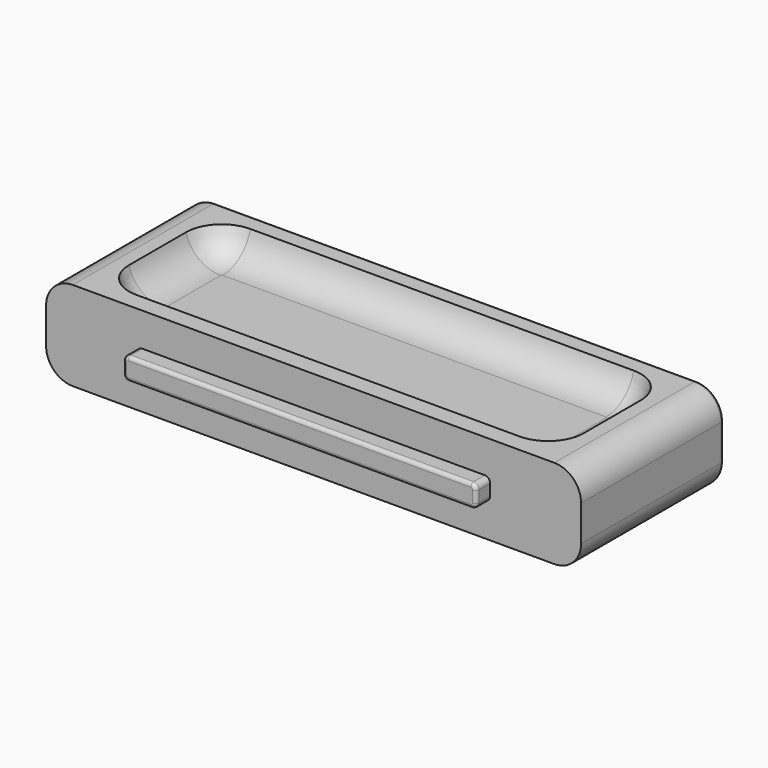
from build123d import *

# Parameters (mm, degrees)
F0_W          = 76.2
F0_H          = 12.7
F1_DEPTH      = 25.4
F2_W          = 50.292
F2_H          = 3.1496
F3_DEPTH      = 2.4892
F4_R          = 0.762
F5_R          = 0.508
F6_R          = 3.81
F7_W          = 64.77
F7_H          = 20.32
F8_DEPTH      = 3.81
F9_R          = 5.08
F10_T1_DEPTH  = 54.61
F10_T3_DEPTH  = 10.16
F10_T6_ANGLE  = 90
F10_T8_ANGLE  = 90
F10_T10_ANGLE = 90
F10_T12_ANGLE = 90
F11_W         = 64.77
F11_H         = 20.32
F12_DEPTH     = 3.81
F13_R         = 5.08
F14_T1_DEPTH  = 54.61
F14_T3_DEPTH  = 10.16
F14_T6_ANGLE  = 90
F14_T8_ANGLE  = 90
F14_T10_ANGLE = 90
F14_T12_ANGLE = 90
F15_R         = 0.508


# Not quite as in the source:
# - a fillet or chamfer that OpenCascade refuses, or shapes differently, is made with other operations: its cross-section is extruded or revolved along the edge and cut away or added


with BuildPart() as f1:
    # F0 (on Front) → F1 (new body)
    with BuildSketch(Plane.XZ):
        Rectangle(F0_W, F0_H)
    extrude(amount=F1_DEPTH)

    # F2 (on face) → F3 (join)
    with BuildSketch(Plane.XZ.offset(25.4)):
        Rectangle(F2_W, F2_H)
    extrude(amount=F3_DEPTH)

    # F4
    f4_edges = [f1.edges().sort_by_distance(p)[0] for p in [
        (-25.146, -26.6446, 1.5748),
        (-25.146, -26.6446, -1.5748),
        (25.146, -26.6446, 1.5748),
        (25.146, -26.6446, -1.5748),
    ]]
    fillet(f4_edges, radius=F4_R)

    # F5
    f5_edges = [f1.edges().sort_by_distance(p)[0] for p in [
        (0, -27.8892, 1.5748),
        (24.922815, -27.8892, 1.351615),
        (-24.922815, -27.8892, 1.351615),
        (25.146, -27.8892, 0),
        (-25.146, -27.8892, 0),
        (24.922815, -27.8892, -1.351615),
        (-24.922815, -27.8892, -1.351615),
        (0, -27.8892, -1.5748),
    ]]
    fillet(f5_edges, radius=F5_R)

    # F6
    f6_edges = [f1.edges().sort_by_distance(p)[0] for p in [
        (38.1, -12.7, 6.35),
        (38.1, -12.7, -6.35),
        (-38.1, -12.7, 6.35),
        (-38.1, -12.7, -6.35),
    ]]
    fillet(f6_edges, radius=F6_R)

    # F7 (on face) → F8 (cut)
    with BuildSketch(Plane.XY.offset(6.35)):
        with Locations((0, -12.7)):
            Rectangle(F7_W, F7_H)
    extrude(amount=-F8_DEPTH, mode=Mode.SUBTRACT)

    # F9
    f9_edges = [f1.edges().sort_by_distance(p)[0] for p in [
        (-32.385, -2.54, 4.445),
        (-32.385, -22.86, 4.445),
        (32.385, -2.54, 4.445),
        (32.385, -22.86, 4.445),
    ]]
    fillet(f9_edges, radius=F9_R)

    # F10: fillet of radius 5.08 on 1 edges, made by hand

    # F10_s2 → F10_t1 (join)
    with BuildSketch(Plane.YZ.offset(-27.305)):
        with BuildLine():
            ThreePointArc((-2.54, 6.35), (-4.3478368763, 3.6039073716), (-7.4586888497, 2.54))
            Line((-7.4586888497, 2.54), (-2.54, 2.54))
            Line((-2.54, 2.54), (-2.54, 6.35))
        make_face()
        with BuildLine():
            ThreePointArc((-22.86, 6.35), (-21.0521631237, 3.6039073716), (-17.9413111503, 2.54))
            Line((-17.9413111503, 2.54), (-22.86, 2.54))
            Line((-22.86, 2.54), (-22.86, 6.35))
        make_face()
    extrude(amount=F10_T1_DEPTH)

    # F10_s4 → F10_t3 (join)
    with BuildSketch(Plane.XZ.offset(7.62)):
        with BuildLine():
            ThreePointArc((-32.385, 6.35), (-30.5771631237, 3.6039073716), (-27.4663111503, 2.54))
            Line((-27.4663111503, 2.54), (-32.385, 2.54))
            Line((-32.385, 2.54), (-32.385, 6.35))
        make_face()
        with BuildLine():
            ThreePointArc((32.385, 6.35), (30.5771631237, 3.6039073716), (27.4663111503, 2.54))
            Line((27.4663111503, 2.54), (32.385, 2.54))
            Line((32.385, 2.54), (32.385, 6.35))
        make_face()
    extrude(amount=F10_T3_DEPTH)

    # F10_s5 → F10_t6 (revolve)
    with BuildSketch(Plane.XZ.offset(7.62)):
        with BuildLine():
            ThreePointArc((32.385, 6.35), (30.5771631237, 3.6039073716), (27.4663111503, 2.54))
            Line((27.4663111503, 2.54), (32.385, 2.54))
            Line((32.385, 2.54), (32.385, 6.35))
        make_face()
    revolve(axis=Axis((27.305, -7.62, 2.54), (0, 0, 1)), revolution_arc=F10_T6_ANGLE)

    # F10_s7 → F10_t8 (revolve)
    with BuildSketch(Plane.XZ.offset(7.62)):
        with BuildLine():
            ThreePointArc((-32.385, 6.35), (-30.5771631237, 3.6039073716), (-27.4663111503, 2.54))
            Line((-27.4663111503, 2.54), (-32.385, 2.54))
            Line((-32.385, 2.54), (-32.385, 6.35))
        make_face()
    revolve(axis=Axis((-27.305, -7.62, 2.54), (0, 0, -1)), revolution_arc=F10_T8_ANGLE)

    # F10_s9 → F10_t10 (revolve)
    with BuildSketch(Plane.YZ.offset(-27.305)):
        with BuildLine():
            ThreePointArc((-22.86, 6.35), (-21.0521631237, 3.6039073716), (-17.9413111503, 2.54))
            Line((-17.9413111503, 2.54), (-22.86, 2.54))
            Line((-22.86, 2.54), (-22.86, 6.35))
        make_face()
    revolve(axis=Axis((-27.305, -17.78, 2.54), (0, 0, -1)), revolution_arc=F10_T10_ANGLE)

    # F10_s11 → F10_t12 (revolve)
    with BuildSketch(Plane.XZ.offset(17.78)):
        with BuildLine():
            ThreePointArc((32.385, 6.35), (30.5771631237, 3.6039073716), (27.4663111503, 2.54))
            Line((27.4663111503, 2.54), (32.385, 2.54))
            Line((32.385, 2.54), (32.385, 6.35))
        make_face()
    revolve(axis=Axis((27.305, -17.78, 2.54), (0, 0, -1)), revolution_arc=F10_T12_ANGLE)

    # F11 (on face) → F12 (cut)
    with BuildSketch(Plane(origin=(0, 0, -6.35), x_dir=(1, 0, 0), z_dir=(0, 0, -1))):
        with Locations((0, 12.7)):
            Rectangle(F11_W, F11_H)
    extrude(amount=-F12_DEPTH, mode=Mode.SUBTRACT)

    # F13
    f13_edges = [f1.edges().sort_by_distance(p)[0] for p in [
        (32.385, -22.86, -4.445),
        (32.385, -2.54, -4.445),
        (-32.385, -22.86, -4.445),
        (-32.385, -2.54, -4.445),
    ]]
    fillet(f13_edges, radius=F13_R)

    # F14: fillet of radius 5.08 on 1 edges, made by hand

    # F14_s2 → F14_t1 (join)
    with BuildSketch(Plane.YZ.offset(-27.305)):
        with BuildLine():
            ThreePointArc((-22.86, -6.35), (-21.0521631237, -3.6039073716), (-17.9413111503, -2.54))
            Line((-17.9413111503, -2.54), (-22.86, -2.54))
            Line((-22.86, -2.54), (-22.86, -6.35))
        make_face()
        with BuildLine():
            ThreePointArc((-2.54, -6.35), (-4.3478368763, -3.6039073716), (-7.4586888497, -2.54))
            Line((-7.4586888497, -2.54), (-2.54, -2.54))
            Line((-2.54, -2.54), (-2.54, -6.35))
        make_face()
    extrude(amount=F14_T1_DEPTH)

    # F14_s4 → F14_t3 (join)
    with BuildSketch(Plane.XZ.offset(7.62)):
        with BuildLine():
            ThreePointArc((32.385, -6.35), (30.5771631237, -3.6039073716), (27.4663111503, -2.54))
            Line((27.4663111503, -2.54), (32.385, -2.54))
            Line((32.385, -2.54), (32.385, -6.35))
        make_face()
        with BuildLine():
            ThreePointArc((-32.385, -6.35), (-30.5771631237, -3.6039073716), (-27.4663111503, -2.54))
            Line((-27.4663111503, -2.54), (-32.385, -2.54))
            Line((-32.385, -2.54), (-32.385, -6.35))
        make_face()
    extrude(amount=F14_T3_DEPTH)

    # F14_s5 → F14_t6 (revolve)
    with BuildSketch(Plane.YZ.offset(27.305)):
        with BuildLine():
            ThreePointArc((-22.86, -6.35), (-21.0521631237, -3.6039073716), (-17.9413111503, -2.54))
            Line((-17.9413111503, -2.54), (-22.86, -2.54))
            Line((-22.86, -2.54), (-22.86, -6.35))
        make_face()
    revolve(axis=Axis((27.305, -17.78, -2.54), (0, 0, 1)), revolution_arc=F14_T6_ANGLE)

    # F14_s7 → F14_t8 (revolve)
    with BuildSketch(Plane.YZ.offset(27.305)):
        with BuildLine():
            ThreePointArc((-2.54, -6.35), (-4.3478368763, -3.6039073716), (-7.4586888497, -2.54))
            Line((-7.4586888497, -2.54), (-2.54, -2.54))
            Line((-2.54, -2.54), (-2.54, -6.35))
        make_face()
    revolve(axis=Axis((27.305, -7.62, -2.54), (0, 0, -1)), revolution_arc=F14_T8_ANGLE)

    # F14_s9 → F14_t10 (revolve)
    with BuildSketch(Plane.YZ.offset(-27.305)):
        with BuildLine():
            ThreePointArc((-2.54, -6.35), (-4.3478368763, -3.6039073716), (-7.4586888497, -2.54))
            Line((-7.4586888497, -2.54), (-2.54, -2.54))
            Line((-2.54, -2.54), (-2.54, -6.35))
        make_face()
    revolve(axis=Axis((-27.305, -7.62, -2.54), (0, 0, 1)), revolution_arc=F14_T10_ANGLE)

    # F14_s11 → F14_t12 (revolve)
    with BuildSketch(Plane.XZ.offset(17.78)):
        with BuildLine():
            ThreePointArc((-32.385, -6.35), (-30.5771631237, -3.6039073716), (-27.4663111503, -2.54))
            Line((-27.4663111503, -2.54), (-32.385, -2.54))
            Line((-32.385, -2.54), (-32.385, -6.35))
        make_face()
    revolve(axis=Axis((-27.305, -17.78, -2.54), (0, 0, 1)), revolution_arc=F14_T12_ANGLE)

    # F15
    f15_edges = [f1.edges().sort_by_distance(p)[0] for p in [
        (-36.984077, 0, 5.234077),
        (0, 0, -6.35),
        (0, 0, 6.35),
        (36.984077, 0, 5.234077),
        (38.1, 0, 0),
        (-38.1, 0, 0),
        (36.984077, 0, -5.234077),
        (-36.984077, 0, -5.234077),
    ]]
    fillet(f15_edges, radius=F15_R)


solid = f1.part
